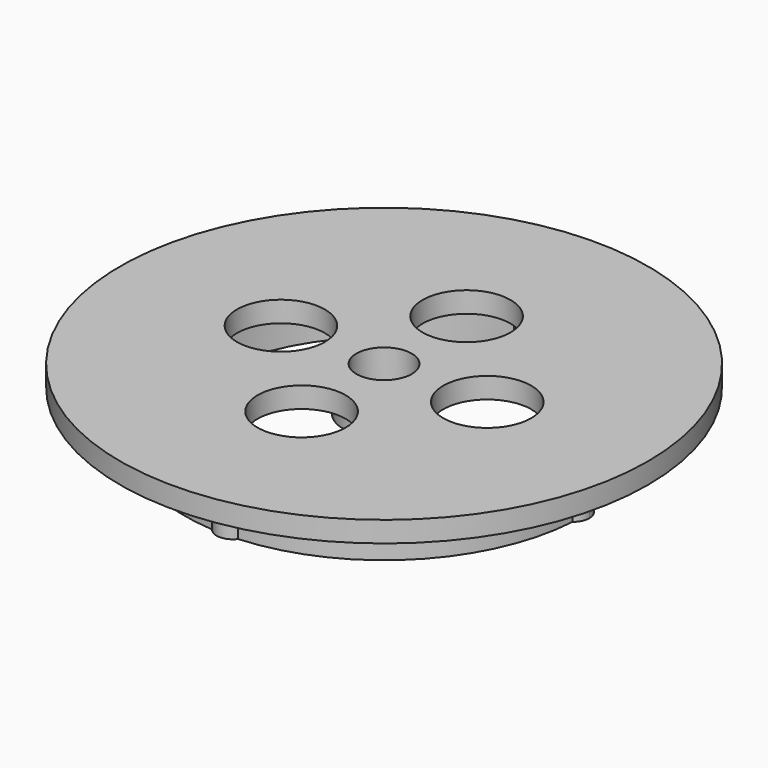
from build123d import *

# Parameters (mm, degrees)
F1_DEPTH = 10
F0_R     = 38.1
F0_R_2   = 6.35
F0_R_3   = 5.8823611715
F2_DEPTH = 3
F0_R_4   = 4
F3_DEPTH = 6.35


with BuildPart() as f1:
    # F0 (on Top) → F1 (new body)
    with BuildSketch(Plane.XY):
        with BuildLine():
            Line((25.7629516235, 0), (28.75, 0))
            ThreePointArc((28.75, 0), (28.7346354423, 0.9398010419), (28.6885581914, 1.878597588))
            ThreePointArc((28.6885581914, 1.878597588), (27.1771412956, 2.3608673988), (25.7015098149, 1.7782209055))
            ThreePointArc((25.7015098149, 1.7782209055), (25.7475865895, 0.889641035), (25.7629516235, 0))
        make_face()
        with BuildLine():
            ThreePointArc((28.6885581914, 1.878597588), (28.7346354423, 0.9398010419), (28.75, 0))
            ThreePointArc((28.75, 0), (28.7346354423, -0.9398010419), (28.6885581914, -1.878597588))
            ThreePointArc((28.6885581914, -1.878597588), (29.3734139116, -1.0481230469), (29.6186758117, 0))
            ThreePointArc((29.6186758117, 0), (29.3734139116, 1.0481230469), (28.6885581914, 1.878597588))
        make_face()
        with BuildLine():
            ThreePointArc((28.6885581914, -1.878597588), (28.7346354423, -0.9398010419), (28.75, 0))
            Line((28.75, 0), (25.7629516235, 0))
            ThreePointArc((25.7629516235, 0), (25.7475865895, -0.889641035), (25.7015098149, -1.7782209055))
            ThreePointArc((25.7015098149, -1.7782209055), (27.1771412956, -2.3608673988), (28.6885581914, -1.878597588))
        make_face()
        with BuildLine():
            ThreePointArc((25.7015098149, 1.7782209055), (27.1771412956, 2.3608673988), (28.6885581914, 1.878597588))
            ThreePointArc((28.6885581914, 1.878597588), (20.3293199591, 20.3293199591), (1.878597588, 28.6885581914))
            ThreePointArc((1.878597588, 28.6885581914), (2.2380361997, 28.0122421835), (2.3622, 27.2564758117))
            ThreePointArc((2.3622, 27.2564758117), (2.2113912208, 26.4259713213), (1.7782209055, 25.7015098149))
            ThreePointArc((1.7782209055, 25.7015098149), (18.2171577963, 18.2171577963), (25.7015098149, 1.7782209055))
        make_face()
        with BuildLine():
            ThreePointArc((1.878597588, -28.6885581914), (20.3293199591, -20.3293199591), (28.6885581914, -1.878597588))
            ThreePointArc((28.6885581914, -1.878597588), (27.1771412956, -2.3608673988), (25.7015098149, -1.7782209055))
            ThreePointArc((25.7015098149, -1.7782209055), (18.2171577963, -18.2171577963), (1.7782209055, -25.7015098149))
            ThreePointArc((1.7782209055, -25.7015098149), (2.2113912208, -26.4259713213), (2.3622, -27.2564758117))
            ThreePointArc((2.3622, -27.2564758117), (2.2380361997, -28.0122421835), (1.878597588, -28.6885581914))
        make_face()
        with BuildLine():
            ThreePointArc((25.7015098149, -1.7782209055), (25.7475865895, -0.889641035), (25.7629516235, 0))
            ThreePointArc((25.7629516235, 0), (25.7475865895, 0.889641035), (25.7015098149, 1.7782209055))
            ThreePointArc((25.7015098149, 1.7782209055), (24.8942758117, 0), (25.7015098149, -1.7782209055))
        make_face()
        with BuildLine():
            ThreePointArc((2.3622, 27.2564758117), (2.2380361997, 28.0122421835), (1.878597588, 28.6885581914))
            ThreePointArc((1.878597588, 28.6885581914), (0.9398010419, 28.7346354423), (0, 28.75))
            Line((0, 28.75), (0, 25.7629516235))
            ThreePointArc((0, 25.7629516235), (0.889641035, 25.7475865895), (1.7782209055, 25.7015098149))
            ThreePointArc((1.7782209055, 25.7015098149), (2.2113912208, 26.4259713213), (2.3622, 27.2564758117))
        make_face()
        with BuildLine():
            ThreePointArc((0, 28.75), (0.9398010419, 28.7346354423), (1.878597588, 28.6885581914))
            ThreePointArc((1.878597588, 28.6885581914), (0, 29.6186758117), (-1.878597588, 28.6885581914))
            ThreePointArc((-1.878597588, 28.6885581914), (-0.9398010419, 28.7346354423), (0, 28.75))
        make_face()
        with BuildLine():
            ThreePointArc((-1.878597588, -28.6885581914), (0, -29.6186758117), (1.878597588, -28.6885581914))
            ThreePointArc((1.878597588, -28.6885581914), (0.9398010419, -28.7346354423), (0, -28.75))
            ThreePointArc((0, -28.75), (-0.9398010419, -28.7346354423), (-1.878597588, -28.6885581914))
        make_face()
        with BuildLine():
            ThreePointArc((0, -28.75), (0.9398010419, -28.7346354423), (1.878597588, -28.6885581914))
            ThreePointArc((1.878597588, -28.6885581914), (2.2380361997, -28.0122421835), (2.3622, -27.2564758117))
            ThreePointArc((2.3622, -27.2564758117), (2.2113912208, -26.4259713213), (1.7782209055, -25.7015098149))
            ThreePointArc((1.7782209055, -25.7015098149), (0.889641035, -25.7475865895), (0, -25.7629516235))
            Line((0, -25.7629516235), (0, -28.75))
        make_face()
        with BuildLine():
            Line((0, 25.7629516235), (0, 28.75))
            ThreePointArc((0, 28.75), (-0.9398010419, 28.7346354423), (-1.878597588, 28.6885581914))
            ThreePointArc((-1.878597588, 28.6885581914), (-2.3608673988, 27.1771412956), (-1.7782209055, 25.7015098149))
            ThreePointArc((-1.7782209055, 25.7015098149), (-0.889641035, 25.7475865895), (0, 25.7629516235))
        make_face()
        with BuildLine():
            ThreePointArc((-1.7782209055, 25.7015098149), (-2.3608673988, 27.1771412956), (-1.878597588, 28.6885581914))
            ThreePointArc((-1.878597588, 28.6885581914), (-20.3293199591, 20.3293199591), (-28.6885581914, 1.878597588))
            ThreePointArc((-28.6885581914, 1.878597588), (-27.1771412956, 2.3608673988), (-25.7015098149, 1.7782209055))
            ThreePointArc((-25.7015098149, 1.7782209055), (-18.2171577963, 18.2171577963), (-1.7782209055, 25.7015098149))
        make_face()
        with BuildLine():
            ThreePointArc((-1.7782209055, 25.7015098149), (0, 24.8942758117), (1.7782209055, 25.7015098149))
            ThreePointArc((1.7782209055, 25.7015098149), (0.889641035, 25.7475865895), (0, 25.7629516235))
            ThreePointArc((0, 25.7629516235), (-0.889641035, 25.7475865895), (-1.7782209055, 25.7015098149))
        make_face()
        with BuildLine():
            ThreePointArc((-1.878597588, -28.6885581914), (-0.9398010419, -28.7346354423), (0, -28.75))
            Line((0, -28.75), (0, -25.7629516235))
            ThreePointArc((0, -25.7629516235), (-0.889641035, -25.7475865895), (-1.7782209055, -25.7015098149))
            ThreePointArc((-1.7782209055, -25.7015098149), (-2.3608673988, -27.1771412956), (-1.878597588, -28.6885581914))
        make_face()
        with BuildLine():
            ThreePointArc((-28.6885581914, -1.878597588), (-20.3293199591, -20.3293199591), (-1.878597588, -28.6885581914))
            ThreePointArc((-1.878597588, -28.6885581914), (-2.3608673988, -27.1771412956), (-1.7782209055, -25.7015098149))
            ThreePointArc((-1.7782209055, -25.7015098149), (-18.2171577963, -18.2171577963), (-25.7015098149, -1.7782209055))
            ThreePointArc((-25.7015098149, -1.7782209055), (-27.1771412956, -2.3608673988), (-28.6885581914, -1.878597588))
        make_face()
        with BuildLine():
            ThreePointArc((0, -25.7629516235), (0.889641035, -25.7475865895), (1.7782209055, -25.7015098149))
            ThreePointArc((1.7782209055, -25.7015098149), (0, -24.8942758117), (-1.7782209055, -25.7015098149))
            ThreePointArc((-1.7782209055, -25.7015098149), (-0.889641035, -25.7475865895), (0, -25.7629516235))
        make_face()
        with BuildLine():
            ThreePointArc((-25.7015098149, 1.7782209055), (-27.1771412956, 2.3608673988), (-28.6885581914, 1.878597588))
            ThreePointArc((-28.6885581914, 1.878597588), (-28.7346354423, 0.9398010419), (-28.75, 0))
            Line((-28.75, 0), (-25.7629516235, 0))
            ThreePointArc((-25.7629516235, 0), (-25.7475865895, 0.889641035), (-25.7015098149, 1.7782209055))
        make_face()
        with BuildLine():
            ThreePointArc((-28.75, 0), (-28.7346354423, 0.9398010419), (-28.6885581914, 1.878597588))
            ThreePointArc((-28.6885581914, 1.878597588), (-29.6186758117, 0), (-28.6885581914, -1.878597588))
            ThreePointArc((-28.6885581914, -1.878597588), (-28.7346354423, -0.9398010419), (-28.75, 0))
        make_face()
        with BuildLine():
            ThreePointArc((-28.75, 0), (-28.7346354423, -0.9398010419), (-28.6885581914, -1.878597588))
            ThreePointArc((-28.6885581914, -1.878597588), (-27.1771412956, -2.3608673988), (-25.7015098149, -1.7782209055))
            ThreePointArc((-25.7015098149, -1.7782209055), (-25.7475865895, -0.889641035), (-25.7629516235, 0))
            Line((-25.7629516235, 0), (-28.75, 0))
        make_face()
        with BuildLine():
            ThreePointArc((-24.8942758117, 0), (-25.1055307267, 0.9764343711), (-25.7015098149, 1.7782209055))
            ThreePointArc((-25.7015098149, 1.7782209055), (-25.7475865895, 0.889641035), (-25.7629516235, 0))
            ThreePointArc((-25.7629516235, 0), (-25.7475865895, -0.889641035), (-25.7015098149, -1.7782209055))
            ThreePointArc((-25.7015098149, -1.7782209055), (-25.1055307267, -0.9764343711), (-24.8942758117, 0))
        make_face()
    extrude(amount=-F1_DEPTH)

    # F0 (on Top) → F2 (join)
    with BuildSketch(Plane.XY):
        Circle(F0_R)
        with BuildLine():
            ThreePointArc((1.878597588, 28.6885581914), (20.3293199591, 20.3293199591), (28.6885581914, 1.878597588))
            ThreePointArc((28.6885581914, 1.878597588), (29.3734139116, 1.0481230469), (29.6186758117, 0))
            ThreePointArc((29.6186758117, 0), (29.3734139116, -1.0481230469), (28.6885581914, -1.878597588))
            ThreePointArc((28.6885581914, -1.878597588), (20.3293199591, -20.3293199591), (1.878597588, -28.6885581914))
            ThreePointArc((1.878597588, -28.6885581914), (0, -29.6186758117), (-1.878597588, -28.6885581914))
            ThreePointArc((-1.878597588, -28.6885581914), (-20.3293199591, -20.3293199591), (-28.6885581914, -1.878597588))
            ThreePointArc((-28.6885581914, -1.878597588), (-29.6186758117, 0), (-28.6885581914, 1.878597588))
            ThreePointArc((-28.6885581914, 1.878597588), (-20.3293199591, 20.3293199591), (-1.878597588, 28.6885581914))
            ThreePointArc((-1.878597588, 28.6885581914), (0, 29.6186758117), (1.878597588, 28.6885581914))
        make_face(mode=Mode.SUBTRACT)
        with BuildLine():
            ThreePointArc((25.7015098149, -1.7782209055), (24.8942758117, 0), (25.7015098149, 1.7782209055))
            ThreePointArc((25.7015098149, 1.7782209055), (18.2171577963, 18.2171577963), (1.7782209055, 25.7015098149))
            ThreePointArc((1.7782209055, 25.7015098149), (0, 24.8942758117), (-1.7782209055, 25.7015098149))
            ThreePointArc((-1.7782209055, 25.7015098149), (-18.2171577963, 18.2171577963), (-25.7015098149, 1.7782209055))
            ThreePointArc((-25.7015098149, 1.7782209055), (-25.1055307267, 0.9764343711), (-24.8942758117, 0))
            ThreePointArc((-24.8942758117, 0), (-25.1055307267, -0.9764343711), (-25.7015098149, -1.7782209055))
            ThreePointArc((-25.7015098149, -1.7782209055), (-18.2171577963, -18.2171577963), (-1.7782209055, -25.7015098149))
            ThreePointArc((-1.7782209055, -25.7015098149), (0, -24.8942758117), (1.7782209055, -25.7015098149))
            ThreePointArc((1.7782209055, -25.7015098149), (18.2171577963, -18.2171577963), (25.7015098149, -1.7782209055))
        make_face()
        with Locations((0, -14.8814758117)):
            Circle(F0_R_2, mode=Mode.SUBTRACT)
        with Locations((-14.8917516235, 0)):
            Circle(F0_R_2, mode=Mode.SUBTRACT)
        Circle(F0_R_3, mode=Mode.SUBTRACT)
        with Locations((14.8917516235, 0)):
            Circle(F0_R_2, mode=Mode.SUBTRACT)
        with Locations((0, 14.8814758117)):
            Circle(F0_R_2, mode=Mode.SUBTRACT)
    extrude(amount=-F2_DEPTH)

    # F0 (on Top) → F3 (join)
    with BuildSketch(Plane.XY):
        Circle(F0_R_3)
        Circle(F0_R_4, mode=Mode.SUBTRACT)
    extrude(amount=-F3_DEPTH)


solid = f1.part
